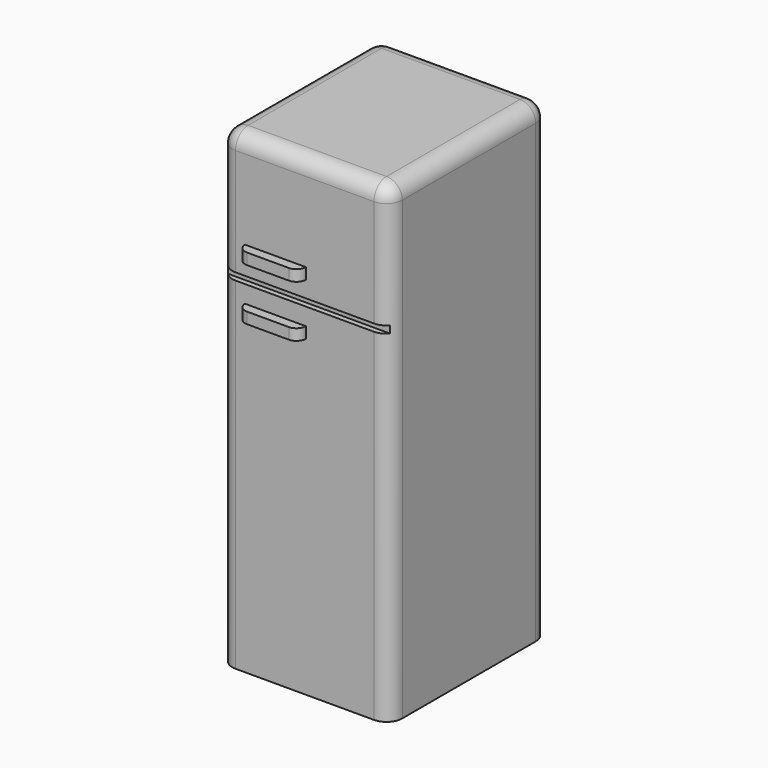
from build123d import *

# Parameters (mm, degrees)
F0_W     = 540
F0_H     = 630
F1_DEPTH = 1500
F2_R     = 50
F3_W     = 42.1213209629
F3_H     = 23.0853557587
F4_DEPTH = 1000
F5_W     = 193.2697791798
F5_H     = 35.2874994278
F6_DEPTH = 30
F7_R     = 29.99999
F7_2_R   = 29.99999


# Not quite as in the source:
# - a fillet or chamfer is up to 0.001 mm smaller than in the source, because OpenCascade refuses the exact size


with BuildPart() as f1:
    # F0 (on Top) → F1 (new body)
    with BuildSketch(Plane.XY):
        with Locations((-13.3859050655, 1.3991128653)):
            Rectangle(F0_W, F0_H)
    extrude(amount=F1_DEPTH)

    # F2
    f2_edges = [f1.edges().sort_by_distance(p)[0] for p in [
        (-13.385905, -313.600887, 1500),
        (-283.385905, 1.399113, 1500),
        (-283.385905, -313.600887, 750),
        (256.614095, -313.600887, 750),
        (256.614095, 1.399113, 1500),
        (256.614095, 316.399113, 750),
        (-13.385905, 316.399113, 1500),
        (-283.385905, 316.399113, 750),
    ]]
    fillet(f2_edges, radius=F2_R)

    # F3 (on face) → F4 (cut)
    with BuildSketch(Plane.YZ.offset(256.6140949345)):
        with Locations((-317.5243586302, 1097.6054668427)):
            Rectangle(F3_W, F3_H)
    extrude(amount=-F4_DEPTH, mode=Mode.SUBTRACT)


with BuildPart() as f6:
    # F5 (on face) → F6 (new body)
    with BuildSketch(Plane.XZ.offset(313.6008871347)):
        with Locations((-106.4450343975, 1178.7065386772)):
            Rectangle(F5_W, F5_H)
    extrude(amount=F6_DEPTH)

    # F7 (radius 30 in the source; OpenCascade refuses exactly that, so slightly less here)
    f7_edges = [f6.edges().sort_by_distance(p)[0] for p in [
        (-203.079924, -343.600887, 1178.706539),
        (-9.810145, -343.600887, 1178.706539),
    ]]
    fillet(f7_edges, radius=F7_R)


with BuildPart() as f6b:
    # F5 (on face) → F6, piece 2 (new body)
    with BuildSketch(Plane.XZ.offset(313.6008871347)):
        with Locations((-106.4450343975, 1013.4190392494)):
            Rectangle(F5_W, F5_H)
    extrude(amount=F6_DEPTH)

    # F7#2 (radius 30 in the source; OpenCascade refuses exactly that, so slightly less here)
    f7_2_edges = [f6b.edges().sort_by_distance(p)[0] for p in [
        (-203.079924, -343.600887, 1013.419039),
        (-9.810145, -343.600887, 1013.419039),
    ]]
    fillet(f7_2_edges, radius=F7_2_R)


solid = Compound([f1.part, f6.part, f6b.part])
